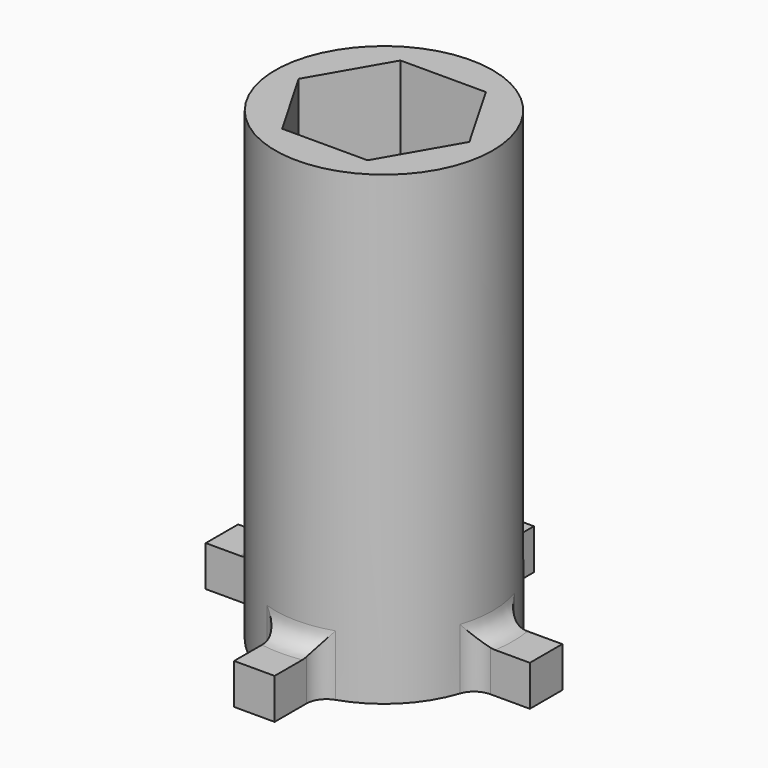
from build123d import *

# Parameters (mm, degrees)
F0_R     = 26.8467875173
F1_DEPTH = 115
F3_DEPTH = 10
F5_R     = 5


# Not quite as in the source:
# - a feature of the source that left no trace in its solid (it failed there, or was rolled back) is left out


with BuildPart() as f1:
    # F0 (on Top) → F1 (new body)
    with BuildSketch(Plane.XY):
        Circle(F0_R)
        Polygon((-21.0732848254, 0), (-10.5366424127, 18.25), (10.5366424127, 18.25), (21.0732848254, 0), (10.5366424127, -18.25), (-10.5366424127, -18.25), align=None, mode=Mode.SUBTRACT)
    extrude(amount=F1_DEPTH)

    # F2 (on Top) → F3 (join)
    with BuildSketch(Plane.XY):
        Polygon((-40, 5), (-40, 0), (-40, -5), (-21.0732848254, -5), (-21.0732848254, 0), (-21.0732848254, 5), align=None)
        Polygon((0, 40), (-5, 40), (-5, 21.0732848254), (0, 21.0732848254), (5, 21.0732848254), (5, 40), align=None)
        Polygon((40, 0), (40, 5), (21.0732848254, 5), (21.0732848254, 0), (21.0732848254, -5), (40, -5), align=None)
        Polygon((0, -40), (5, -40), (5, -21.0732848254), (0, -21.0732848254), (-5, -21.0732848254), (-5, -40), align=None)
    extrude(amount=F3_DEPTH)

    # F5
    f5_edges = [f1.edges().sort_by_distance(p)[0] for p in [
        (0, 26.846788, 10),
        (-26.846788, 0, 10),
        (0, -26.846788, 10),
        (26.729101, 2.511007, 10),
        (26.729101, -2.511007, 10),
        (26.377073, -5, 5),
        (5, -26.377073, 5),
        (-5, -26.377073, 5),
        (-26.377073, -5, 5),
        (-26.377073, 5, 5),
        (-5, 26.377073, 5),
        (5, 26.377073, 5),
        (26.377073, 5, 5),
    ]]
    fillet(f5_edges, radius=F5_R)


solid = f1.part
